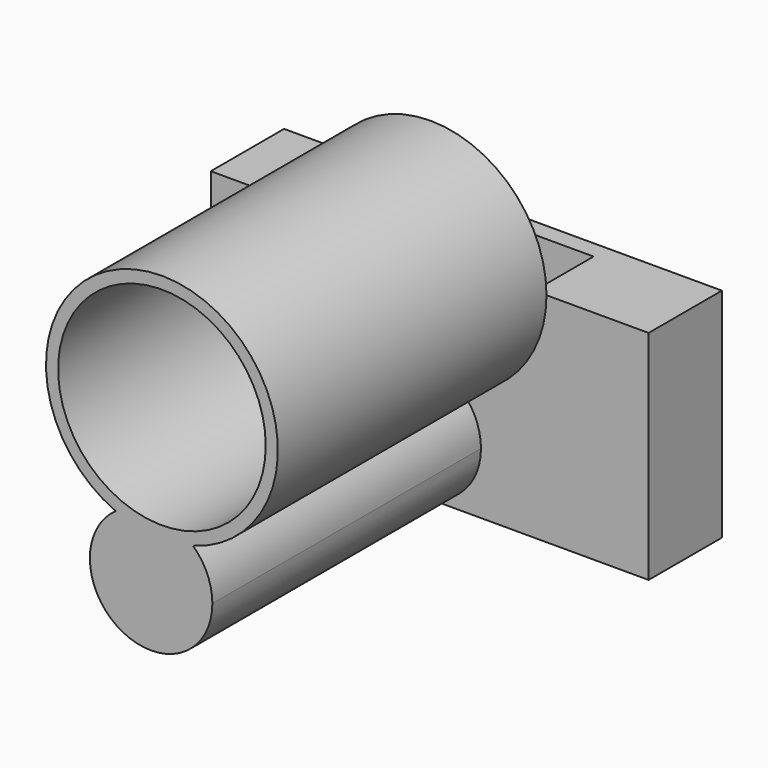
from build123d import *

# Parameters (mm, degrees)
F0_R     = 40.1716956085
F1_DEPTH = 116.332
F2_R     = 35.9669846415
F3_DEPTH = 116.333
F5_DEPTH = 31.75
F6_DEPTH = 25.654
F8_DEPTH = 116.332


with BuildPart() as f1:
    # F0 (on Front) → F1 (new body)
    with BuildSketch(Plane.XZ):
        Circle(F0_R)
    extrude(amount=F1_DEPTH)

    # F2 (on face) → F3 (cut, through all)
    with BuildSketch(Plane.XZ.offset(116.332)):
        Circle(F2_R)
    extrude(amount=-F3_DEPTH, mode=Mode.SUBTRACT)

    # F4 (on Front) → F5 (join)
    with BuildSketch(Plane.XZ):
        Polygon((75.5550265312, 0), (0, 0), (-75.4067823291, 0), (-76.1463865638, 0), (-76.1463865638, -75.3481909633), (75.5550265312, -75.3481909633), align=None)
    extrude(amount=-F5_DEPTH)

    # F6 (cut): a face of the model
    f6_faces = [f1.faces().sort_by_distance(p)[0] for p in [
        (0, 0, -15.2648623835),
    ]]
    extrude(f6_faces, amount=-F6_DEPTH, mode=Mode.SUBTRACT)

    # F7 (on face) → F8 (join)
    with BuildSketch(Plane.XZ):
        with BuildLine():
            ThreePointArc((-3.7476888392, -75.3481909633), (11.2568342092, -69.1331140197), (17.4719111528, -54.1285909712))
            ThreePointArc((17.4719111528, -54.1285909712), (15.7353214008, -45.7212289706), (10.8097935034, -38.6899663024))
            ThreePointArc((10.8097935034, -38.6899663024), (-2.7747158074, -40.0757542693), (-16.0386260655, -36.8310684341))
            ThreePointArc((-16.0386260655, -36.8310684341), (-23.9630039853, -60.5793628138), (-3.7476888392, -75.3481909633))
        make_face()
    extrude(amount=F8_DEPTH)


solid = f1.part
